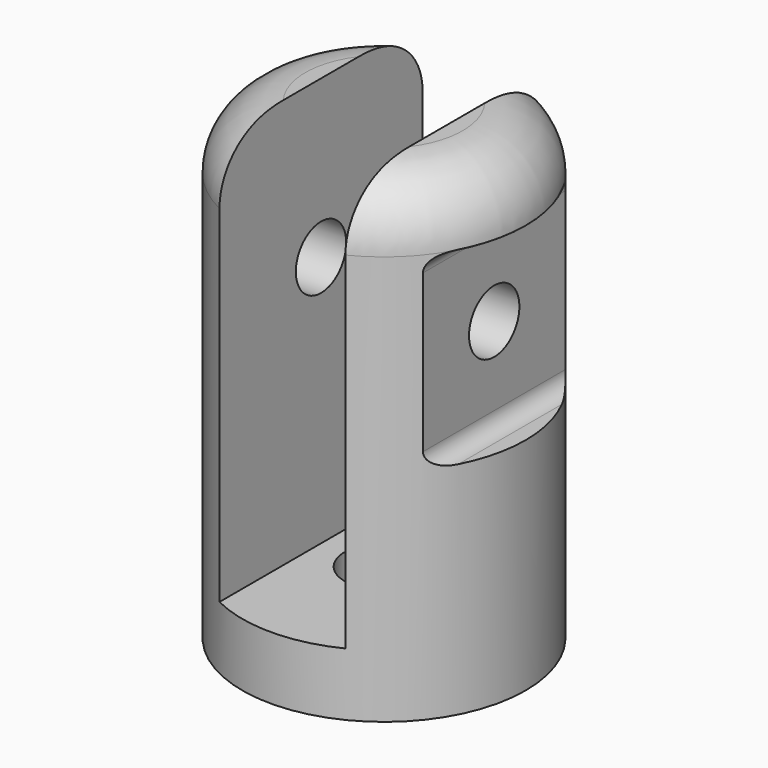
from build123d import *

# Parameters (mm, degrees)
F0_R          = 45
F0_R_2        = 12.5
F1_DEPTH      = 150
F2_W          = 40
F2_H          = 150
F2_W_2        = 22.3551505804
F2_H_2        = 60
F3_DEPTH      = 100
F3_DEPTH_BACK = 100
F4_R          = 19.99999
F5_R          = 5
F6_R          = 10
F7_DEPTH      = 150


# Not quite as in the source:
# - a fillet or chamfer is up to 0.001 mm smaller than in the source, because OpenCascade refuses the exact size


with BuildPart() as f1:
    # F0 (on Top) → F1 (new body)
    with BuildSketch(Plane.XY):
        Circle(F0_R)
        Circle(F0_R_2, mode=Mode.SUBTRACT)
    extrude(amount=F1_DEPTH)

    # F2 (on Front) → F3 (cut, two sides)
    with BuildSketch(Plane.XZ) as f3_sk:
        with Locations((0, 95)):
            Rectangle(F2_W, F2_H)
        with Locations((-46.1775752902, 100)):
            Rectangle(F2_W_2, F2_H_2)
        with Locations((46.1775752902, 100)):
            Rectangle(F2_W_2, F2_H_2)
    extrude(amount=-F3_DEPTH, mode=Mode.SUBTRACT)
    extrude(f3_sk.sketch, amount=F3_DEPTH_BACK, mode=Mode.SUBTRACT)

    # F4 (radius 20 in the source; OpenCascade refuses exactly that, so slightly less here)
    f4_edges = [f1.edges().sort_by_distance(p)[0] for p in [
        (-45, 0, 150),
        (38.242646, -23.717082, 150),
        (38.242646, 23.717082, 150),
    ]]
    fillet(f4_edges, radius=F4_R)

    # F5
    f5_edges = [f1.edges().sort_by_distance(p)[0] for p in [
        (-35, 0, 130),
        (-35, 0, 70),
        (35, 0, 70),
        (35, 0, 130),
    ]]
    fillet(f5_edges, radius=F5_R)

    # F6 (on face) → F7 (cut)
    with BuildSketch(Plane.YZ.offset(35)):
        with Locations((0, 100)):
            Circle(F6_R)
    extrude(amount=-F7_DEPTH, mode=Mode.SUBTRACT)


solid = f1.part
